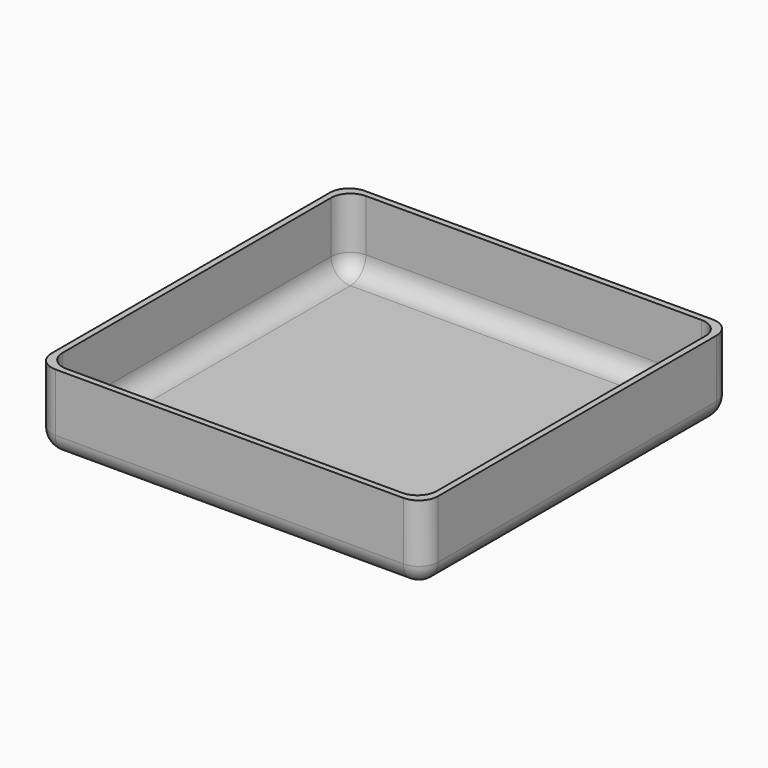
from build123d import *

# Parameters (mm, degrees)
F0_W         = 100
F0_H         = 100
F1_DEPTH     = 20
F2_T         = -1.6
F3_R         = 5
F4_T1_DEPTH  = 13.4
F4_S5_W      = 5
F4_S5_H      = 5
F4_T6_DEPTH  = 5
F4_S11_W     = 5
F4_S11_H     = 5
F4_T12_DEPTH = 5
F4_S17_W     = 5
F4_S17_H     = 5
F4_T18_DEPTH = 5
F4_S23_W     = 5
F4_S23_H     = 5
F4_T24_DEPTH = 5
F5_R         = 5
F6_R         = 5


# Not quite as in the source:
# - a fillet or chamfer that OpenCascade refuses, or shapes differently, is made with other operations: its cross-section is extruded or revolved along the edge and cut away or added


with BuildPart() as f1:
    # F0 (on Top) → F1 (new body)
    with BuildSketch(Plane.XY):
        Rectangle(F0_W, F0_H)
    extrude(amount=F1_DEPTH)

    # F2
    f2_openings = [f1.faces().sort_by_distance(p)[0] for p in [
        (0, 0, 20),
    ]]
    offset(amount=F2_T, openings=f2_openings)

    # F3
    f3_edges = [f1.edges().sort_by_distance(p)[0] for p in [
        (-48.4, 0, 1.6),
        (0, 48.4, 1.6),
        (48.4, 0, 1.6),
        (0, -48.4, 1.6),
    ]]
    fillet(f3_edges, radius=F3_R)

    # F4: fillet of radius 5 on 8 edges, made by hand

    # F4_s2 → F4_t1 (join)
    with BuildSketch(Plane.XY.offset(6.6)):
        with BuildLine():
            ThreePointArc((43.4, 48.4), (46.9355339059, 46.9355339059), (48.4, 43.4))
            Line((48.4, 43.4), (48.4, 48.4))
            Line((48.4, 48.4), (43.4, 48.4))
        make_face()
        with BuildLine():
            ThreePointArc((48.4, -43.4), (46.9355339059, -46.9355339059), (43.4, -48.4))
            Line((43.4, -48.4), (48.4, -48.4))
            Line((48.4, -48.4), (48.4, -43.4))
        make_face()
        with BuildLine():
            ThreePointArc((-48.4, -43.4), (-46.9355339059, -46.9355339059), (-43.4, -48.4))
            Line((-43.4, -48.4), (-48.4, -48.4))
            Line((-48.4, -48.4), (-48.4, -43.4))
        make_face()
        with BuildLine():
            ThreePointArc((-43.4, 48.4), (-46.9355339059, 46.9355339059), (-48.4, 43.4))
            Line((-48.4, 43.4), (-48.4, 48.4))
            Line((-48.4, 48.4), (-43.4, 48.4))
        make_face()
    extrude(amount=F4_T1_DEPTH)


with BuildPart() as f4_tool4:
    # F4_s5 → F4_t6 (new body)
    with BuildSketch(Plane.XZ.offset(-43.4)):
        with Locations((45.9, 4.1)):
            Rectangle(F4_S5_W, F4_S5_H)
    extrude(amount=-F4_T6_DEPTH)

    # F4_s7 → F4_t8 (revolve, cut)
    with BuildSketch(Plane(origin=(43.4, 43.4, 6.6), x_dir=(-0.7071067812, 0, 0.7071067812), z_dir=(-0.7071067812, 0, -0.7071067812))):
        with BuildLine():
            ThreePointArc((0, -5), (5, 0), (0, 5))
            Line((0, 5), (0, -5))
        make_face()
    revolve(axis=Axis((43.4, 43.4, 6.6), (0, 1, 0)), mode=Mode.SUBTRACT)


with BuildPart() as f1_1:
    add(f1.part)

    # F4_t3: union F4_tool4
    add(f4_tool4.part)


with BuildPart() as f4_tool10:
    # F4_s11 → F4_t12 (new body)
    with BuildSketch(Plane.YZ.offset(43.4)):
        with Locations((-45.9, 4.1)):
            Rectangle(F4_S11_W, F4_S11_H)
    extrude(amount=F4_T12_DEPTH)

    # F4_s13 → F4_t14 (revolve, cut)
    with BuildSketch(Plane(origin=(43.4, -43.4, 6.6), x_dir=(0, 0.7071067812, 0.7071067812), z_dir=(0, 0.7071067812, -0.7071067812))):
        with BuildLine():
            ThreePointArc((0, -5), (5, 0), (0, 5))
            Line((0, 5), (0, -5))
        make_face()
    revolve(axis=Axis((43.4, -43.4, 6.6), (1, 0, 0)), mode=Mode.SUBTRACT)


with BuildPart() as f1_2:
    add(f1_1.part)

    # F4_t9: union F4_tool10
    add(f4_tool10.part)


with BuildPart() as f4_tool16:
    # F4_s17 → F4_t18 (new body)
    with BuildSketch(Plane.YZ.offset(-43.4)):
        with Locations((-45.9, 4.1)):
            Rectangle(F4_S17_W, F4_S17_H)
    extrude(amount=-F4_T18_DEPTH)

    # F4_s19 → F4_t20 (revolve, cut)
    with BuildSketch(Plane(origin=(-43.4, -43.4, 6.6), x_dir=(0, 0.7071067812, 0.7071067812), z_dir=(0, -0.7071067812, 0.7071067812))):
        with BuildLine():
            ThreePointArc((0, -5), (5, 0), (0, 5))
            Line((0, 5), (0, -5))
        make_face()
    revolve(axis=Axis((-43.4, -43.4, 6.6), (-1, 0, 0)), mode=Mode.SUBTRACT)


with BuildPart() as f1_3:
    add(f1_2.part)

    # F4_t15: union F4_tool16
    add(f4_tool16.part)


with BuildPart() as f4_tool22:
    # F4_s23 → F4_t24 (new body)
    with BuildSketch(Plane.XZ.offset(-43.4)):
        with Locations((-45.9, 4.1)):
            Rectangle(F4_S23_W, F4_S23_H)
    extrude(amount=-F4_T24_DEPTH)

    # F4_s25 → F4_t26 (revolve, cut)
    with BuildSketch(Plane(origin=(-43.4, 43.4, 6.6), x_dir=(0.7071067812, 0, 0.7071067812), z_dir=(-0.7071067812, 0, 0.7071067812))):
        with BuildLine():
            ThreePointArc((0, -5), (5, 0), (0, 5))
            Line((0, 5), (0, -5))
        make_face()
    revolve(axis=Axis((-43.4, 43.4, 6.6), (0, 1, 0)), mode=Mode.SUBTRACT)


with BuildPart() as f1_4:
    add(f1_3.part)

    # F4_t21: union F4_tool22
    add(f4_tool22.part)

    # F5
    f5_edges = [f1_4.edges().sort_by_distance(p)[0] for p in [
        (50, -50, 10),
        (-50, -50, 10),
        (-50, 50, 10),
        (50, 50, 10),
    ]]
    fillet(f5_edges, radius=F5_R)

    # F6
    f6_edges = [f1_4.edges().sort_by_distance(p)[0] for p in [
        (-50, 0, 0),
        (0, 50, 0),
        (-48.535534, 48.535534, 0),
        (48.535534, 48.535534, 0),
        (50, 0, 0),
        (48.535534, -48.535534, 0),
        (0, -50, 0),
        (-48.535534, -48.535534, 0),
    ]]
    fillet(f6_edges, radius=F6_R)


solid = f1_4.part
